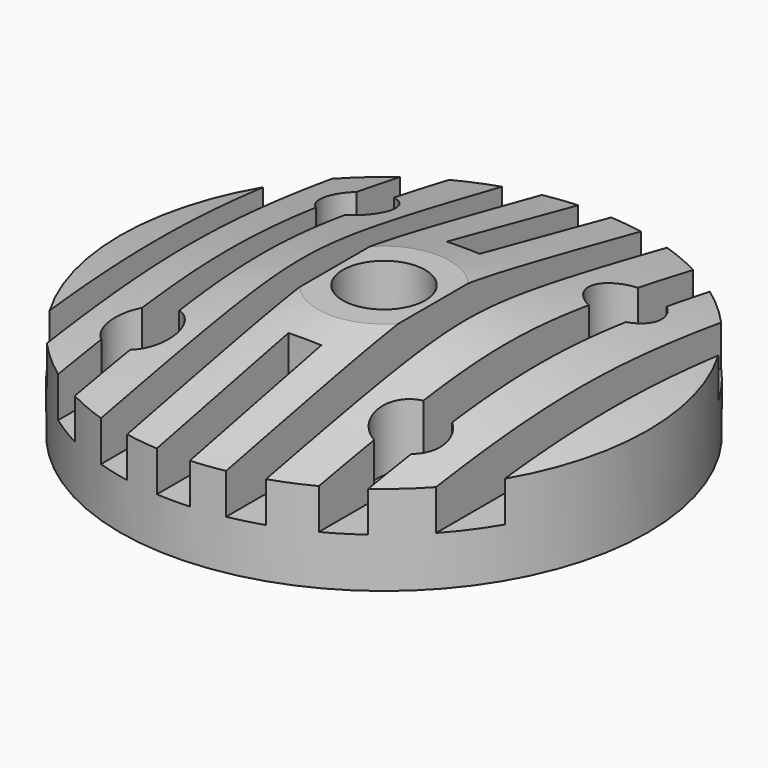
from build123d import *

# Parameters (mm, degrees)
F3_D            = 3
F3_CBORE_D      = 5
F3_CBORE_DEPTH  = 4
F4_D            = 2.5
F4_CBORE_D      = 4
F4_CBORE_DEPTH  = 5
F4_COPIES_COUNT = 4
F5_W            = 2
F5_H            = 35
F5_H_2          = 11.5
F6_DEPTH        = 5


# Not quite as in the source:
# - a pattern or mirror of a feature is missing from the dataset's text; its kind, count and spacing are read off the source's solid


with BuildPart() as f1:
    # F0 (on Front) → F1 (revolve)
    with BuildSketch(Plane.XZ):
        Polygon((0, 8), (0, 0), (8, 0), (8, -1), (9, -1), (9, 0), (16, 0), (16, 5.44932126), (4, 8), align=None)
    revolve(axis=Axis((0, 0, 4), (0, 0, 1)))

    # F3 (through all)
    with Locations(Plane.XY.offset(8)):
        with Locations((0, 0)):
            CounterBoreHole(F3_D / 2, F3_CBORE_D / 2, F3_CBORE_DEPTH)

    # F4 (through all)
    with Locations(Plane.XY.offset(8)):
        with Locations((-8.1317279836, 8.1317279836)):
            f4 = CounterBoreHole(F4_D / 2, F4_CBORE_D / 2, F4_CBORE_DEPTH)

    # F4_copies: F4 ×4 about axis
    f4_copies_axis = Axis((0, 0, 0), (0, 0, 1))
    for i in range(1, F4_COPIES_COUNT):
        add(f4.rotate(f4_copies_axis, i * 360 / F4_COPIES_COUNT), mode=Mode.SUBTRACT)

    # F5 (on face) → F6 (cut)
    with BuildSketch(Plane.XY.offset(8)):
        with Locations((-4, 0)):
            Rectangle(F5_W, F5_H)
        with Locations((-8.4, 0)):
            Rectangle(F5_W, F5_H)
        with Locations((-12.8, 0)):
            Rectangle(F5_W, F5_H)
        with Locations((4, 0)):
            Rectangle(F5_W, F5_H)
        with Locations((8.4, 0)):
            Rectangle(F5_W, F5_H)
        with Locations((12.8, 0)):
            Rectangle(F5_W, F5_H)
        with Locations((0, 11.75)):
            Rectangle(F5_W, F5_H_2)
        with Locations((0, -11.75)):
            Rectangle(F5_W, F5_H_2)
    extrude(amount=-F6_DEPTH, mode=Mode.SUBTRACT)


solid = f1.part
